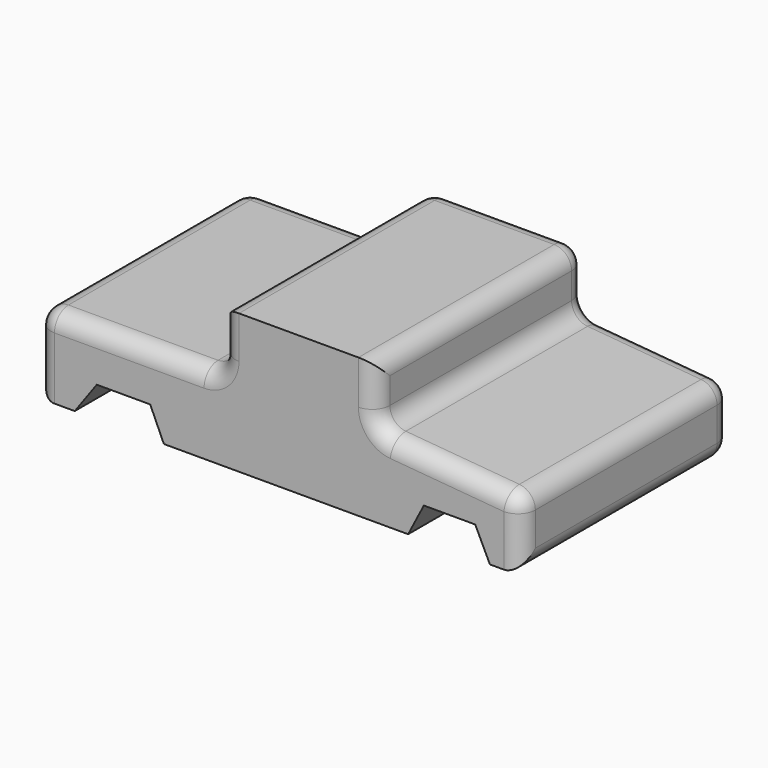
from build123d import *

# Parameters (mm, degrees)
F1_DEPTH = 38.1
F2_R     = 5.08


with BuildPart() as f1:
    # F0 (on Front) → F1 (new body, symmetric)
    with BuildSketch(Plane.XZ):
        Polygon((-44.8818020523, 10.0584002212), (-98.5266044736, 10.0584002212), (-98.5266044736, -13.1064001471), (-87.5537991524, -13.1064001471), (-81.152997911, -4.2672003619), (-65.6082034111, -4.2672003619), (-61.6458021104, -13.1064001471), (9.3726003543, -13.1064001471), (13.9445997775, -4.2672003619), (28.8797989488, -4.2672003619), (33.1469997764, -13.1064001471), (42.2910004854, -13.1064001471), (42.2910004854, 6.4007998444), (0, 10.0584002212), (0, 27.4320002645), (-44.8818020523, 27.4320002645), align=None)
    extrude(amount=F1_DEPTH, both=True)

    # F2
    f2_edges = [f1.edges().sort_by_distance(p)[0] for p in [
        (21.412199, 38.1, -4.2672),
        (31.013399, 38.1, -8.6868),
        (37.719, 38.1, -13.1064),
        (42.291, 38.1, -3.3528),
        (21.1455, 38.1, 8.2296),
        (0, 38.1, 18.7452),
        (-22.440901, 38.1, 27.432),
        (-44.881802, 38.1, 18.7452),
        (-71.704203, 38.1, 10.0584),
        (-98.526604, 38.1, -1.524),
        (-93.040202, 38.1, -13.1064),
        (-84.353399, 38.1, -8.6868),
        (-73.380601, 38.1, -4.2672),
        (-63.627003, 38.1, -8.6868),
        (-26.136601, 38.1, -13.1064),
        (11.6586, 38.1, -8.6868),
        (-98.526604, 0, 10.0584),
        (-98.526604, 0, -13.1064),
        (-98.526604, -38.1, -1.524),
        (-44.881802, 0, 27.432),
        (-44.881802, 0, 10.0584),
        (-44.881802, -38.1, 18.7452),
        (0, 0, 10.0584),
        (0, 0, 27.432),
        (0, -38.1, 18.7452),
        (42.291, 0, -13.1064),
        (42.291, 0, 6.4008),
        (42.291, -38.1, -3.3528),
        (-71.704203, -38.1, 10.0584),
        (21.1455, -38.1, 8.2296),
    ]]
    fillet(f2_edges, radius=F2_R)


solid = f1.part
